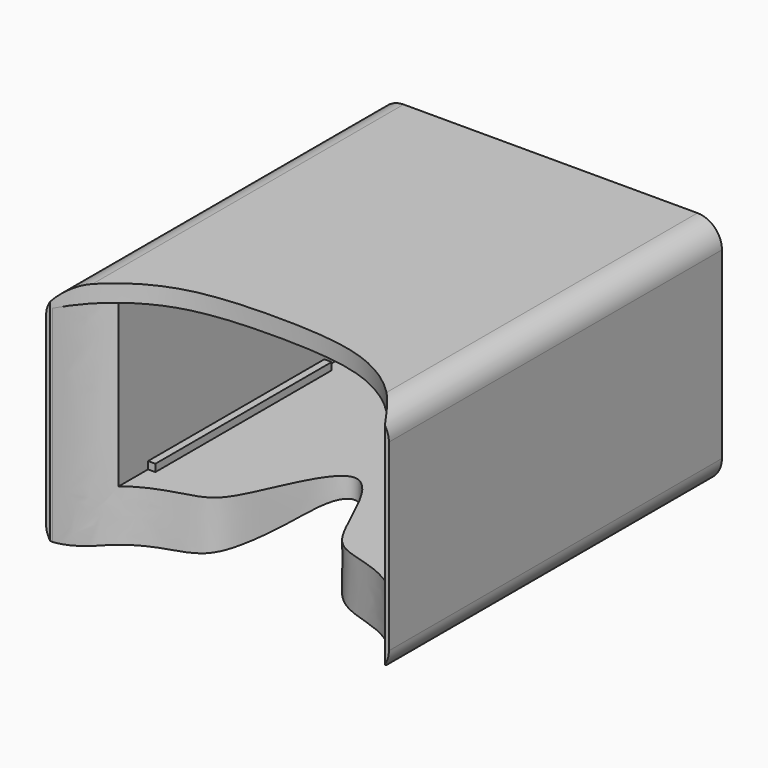
from build123d import *

# Parameters (mm, degrees)
F0_W      = 140
F0_H      = 170
F1_DEPTH  = 95
F2_W      = 110
F2_H      = 67
F3_DEPTH  = 170.001
F5_DEPTH  = 88
F7_DEPTH  = 95.001
F8_R      = 10
F10_DEPTH = 170.001
F11_W     = 121
F11_H     = 76
F11_W_2   = 110
F11_H_2   = 67
F12_DEPTH = 3
F13_W     = 3
F13_H     = 90
F14_DEPTH = 3
F15_W     = 3
F15_H     = 90
F16_DEPTH = 3
F17_R     = 1.3
F18_DEPTH = 100
F19_R     = 3.1
F20_DEPTH = 75


with BuildPart() as f1:
    # F0 (on Top) → F1 (new body)
    with BuildSketch(Plane.XY):
        Rectangle(F0_W, F0_H)
    extrude(amount=F1_DEPTH)

    # F2 (on face) → F3 (cut, through all)
    with BuildSketch(Plane.XZ.offset(85)):
        with Locations((0, 54.5)):
            Rectangle(F2_W, F2_H)
    extrude(amount=-F3_DEPTH, mode=Mode.SUBTRACT)

    # F4 (on face) → F5 (cut)
    with BuildSketch(Plane(origin=(0, 0, 0), x_dir=(1, 0, 0), z_dir=(0, 0, -1))):
        with BuildLine():
            add(Edge.make_bspline(
                [(0, 15), (-7.79441, 15), (-19.466411, 48.056936), (-30.975012, 59.107625), (-57.856268, 61.12551), (-68.258241, 85)],
                knots=[0, 0, 0, 0, 0.355883, 0.597297, 1, 1, 1, 1], degree=3))
            add(Edge.make_bspline(
                [(0, 15), (7.79441, 15), (19.466411, 48.056936), (30.975012, 59.107625), (57.856268, 61.12551), (68.258241, 85)],
                knots=[0, 0, 0, 0, 0.355883, 0.597297, 1, 1, 1, 1], degree=3))
            Line((68.258241, 85), (-68.258241, 85))
        make_face()
    extrude(amount=-F5_DEPTH, mode=Mode.SUBTRACT)

    # F6 (on face) → F7 (cut, through all)
    with BuildSketch(Plane.XY.offset(95)):
        with BuildLine():
            add(Edge.make_bspline(
                [(0, -55), (25.389496, -55), (47.041007, -60.614282), (62.843867, -75.413413), (68.355819, -85)],
                knots=[0, 0, 0, 0, 0.564508, 1, 1, 1, 1], degree=3))
            add(Edge.make_bspline(
                [(0, -55), (-25.389496, -55), (-47.041007, -60.614282), (-62.843867, -75.413413), (-68.355819, -85)],
                knots=[0, 0, 0, 0, 0.564508, 1, 1, 1, 1], degree=3))
            Line((-68.355819, -85), (68.355819, -85))
        make_face()
    extrude(amount=-F7_DEPTH, mode=Mode.SUBTRACT)

    # F8
    f8_edges = [f1.edges().sort_by_distance(p)[0] for p in [
        (70, 0, 95),
        (70, 0, 0),
        (-70, 0, 0),
        (-70, 0, 95),
    ]]
    fillet(f8_edges, radius=F8_R)

    # F9 (on face) → F10 (cut, through all)
    with BuildSketch(Plane(origin=(0, 85, 0), x_dir=(-1, 0, 0), z_dir=(0, 1, 0))):
        with BuildLine():
            add(Edge.make_bspline(
                [(0, 13), (14.179069, 13), (11.016984, 0), (40, 0)],
                knots=[0, 0, 0, 0, 42.059482, 42.059482, 42.059482, 42.059482], degree=3))
            add(Edge.make_bspline(
                [(0, 13), (-14.179069, 13), (-11.016984, 0), (-40, 0)],
                knots=[0, 0, 0, 0, 42.059482, 42.059482, 42.059482, 42.059482], degree=3))
            Line((-40, 0), (40, 0))
        make_face()
    extrude(amount=-F10_DEPTH, mode=Mode.SUBTRACT)

    # F11 (on face) → F12 (cut)
    with BuildSketch(Plane(origin=(0, 85, 0), x_dir=(-1, 0, 0), z_dir=(0, 1, 0))):
        with Locations((0, 52)):
            Rectangle(F11_W, F11_H)
        with Locations((0, 54.5)):
            Rectangle(F11_W_2, F11_H_2, mode=Mode.SUBTRACT)
    extrude(amount=-F12_DEPTH, mode=Mode.SUBTRACT)

    # F13 (on face) → F14 (join)
    with BuildSketch(Plane.XY.offset(21)):
        with Locations((-53.5, -6.706829)):
            Rectangle(F13_W, F13_H)
        with Locations((53.5, -6.706829)):
            Rectangle(F13_W, F13_H)
    extrude(amount=F14_DEPTH)

    # F15 (on face) → F16 (join)
    with BuildSketch(Plane(origin=(0, 0, 88), x_dir=(1, 0, 0), z_dir=(0, 0, -1))):
        with Locations((53.5, 6.706829)):
            Rectangle(F15_W, F15_H)
        with Locations((-53.5, 6.706829)):
            Rectangle(F15_W, F15_H)
    extrude(amount=F16_DEPTH)

    # F17 (on face) → F18 (cut)
    with BuildSketch(Plane(origin=(0, 85, 0), x_dir=(-1, 0, 0), z_dir=(0, 1, 0))):
        with Locations((65, 77.5)):
            Circle(F17_R)
        with Locations((65, 17.5)):
            Circle(F17_R)
        with Locations((-65, 77.5)):
            Circle(F17_R)
        with Locations((-65, 17.5)):
            Circle(F17_R)
    extrude(amount=-F18_DEPTH, mode=Mode.SUBTRACT)

    # F19 (on face) → F20 (cut)
    with BuildSketch(Plane(origin=(0, 85, 0), x_dir=(-1, 0, 0), z_dir=(0, 1, 0))):
        with Locations((65, 77.5)):
            Circle(F19_R)
        with Locations((65, 17.5)):
            Circle(F19_R)
        with Locations((-65, 77.5)):
            Circle(F19_R)
        with Locations((-65, 17.5)):
            Circle(F19_R)
    extrude(amount=-F20_DEPTH, mode=Mode.SUBTRACT)


solid = f1.part
